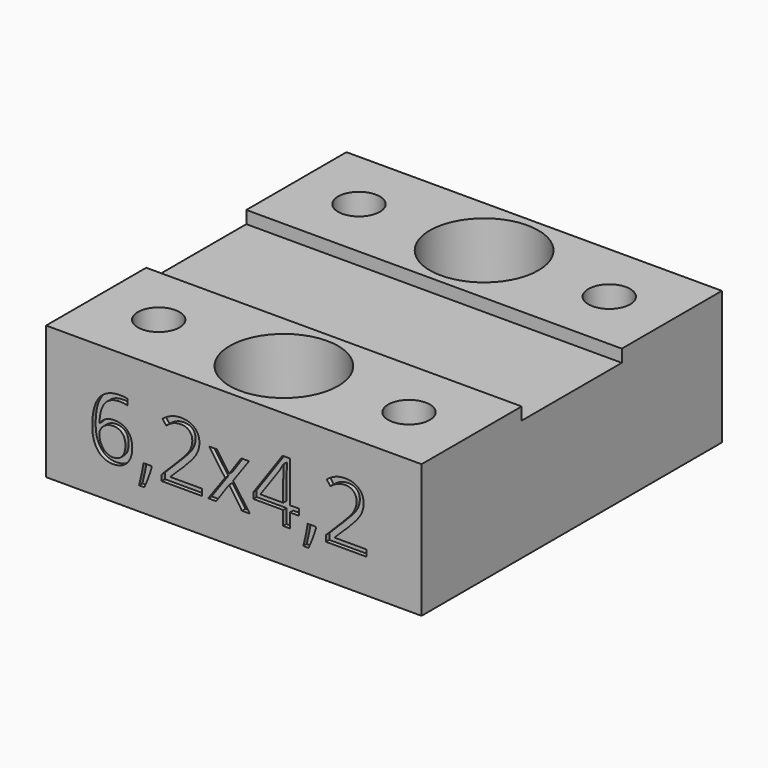
from build123d import *

# Parameters (mm, degrees)
F1_DEPTH     = 90
F2_R         = 5
F2_R_2       = 13
F3_DEPTH     = 32
F4_R         = 13
F5_DEPTH     = 25
F6_TEXT_SIZE = 20.5860020489
F7_DEPTH     = 1


# Not quite as in the source:
# - Text() gives the source's letters only with a copy of the font that has no kerning and outlines rounded to 1/6400 em; it was checked with that copy


with BuildPart() as f1:
    # F0 (on Right) → F1 (new body)
    with BuildSketch(Plane.YZ):
        Polygon((-46.9016340375, 12.252841084), (-46.9016340375, -19.747158916), (43.0983659625, -19.747158916), (43.0983659625, 12.252841084), (13.0983659625, 12.252841084), (13.0983659625, 9.252841084), (-16.9016340375, 9.252841084), (-16.9016340375, 12.252841084), align=None)
    extrude(amount=F1_DEPTH)

    # F2 (on face) → F3 (cut, through all)
    with BuildSketch(Plane.XY.offset(12.252841084)):
        with Locations((15, 28.0983659625)):
            Circle(F2_R)
        with Locations((75, 28.0983659625)):
            Circle(F2_R)
        with Locations((15, -31.9016340375)):
            Circle(F2_R)
        with Locations((75, -31.9016340375)):
            Circle(F2_R)
        with Locations((45, 28.0983659625)):
            Circle(F2_R_2)
        with Locations((45, -31.9016340375)):
            Circle(F2_R_2)
    extrude(amount=-F3_DEPTH, mode=Mode.SUBTRACT)

    # F4 (on face) → F5 (cut)
    with BuildSketch(Plane(origin=(0, 0, -19.747158916), x_dir=(1, 0, 0), z_dir=(0, 0, -1))):
        with Locations((15, 31.9016340374)):
            Circle(F4_R)
        with Locations((75, 31.9016340374)):
            Circle(F4_R)
        with Locations((15, -28.0983659626)):
            Circle(F4_R)
        with Locations((75, -28.0983659626)):
            Circle(F4_R)
    extrude(amount=-F5_DEPTH, mode=Mode.SUBTRACT)

    # F6 (on face) → F7 (cut)
    with BuildSketch(Plane.XZ.offset(46.9016340375)):
        with Locations((9.8924310878, -11.566551053)):
            Text('6,2x4,2', F6_TEXT_SIZE, font='Open Sans', text_align=(TextAlign.LEFT, TextAlign.BOTTOM))
    extrude(amount=-F7_DEPTH, mode=Mode.SUBTRACT)


solid = f1.part
